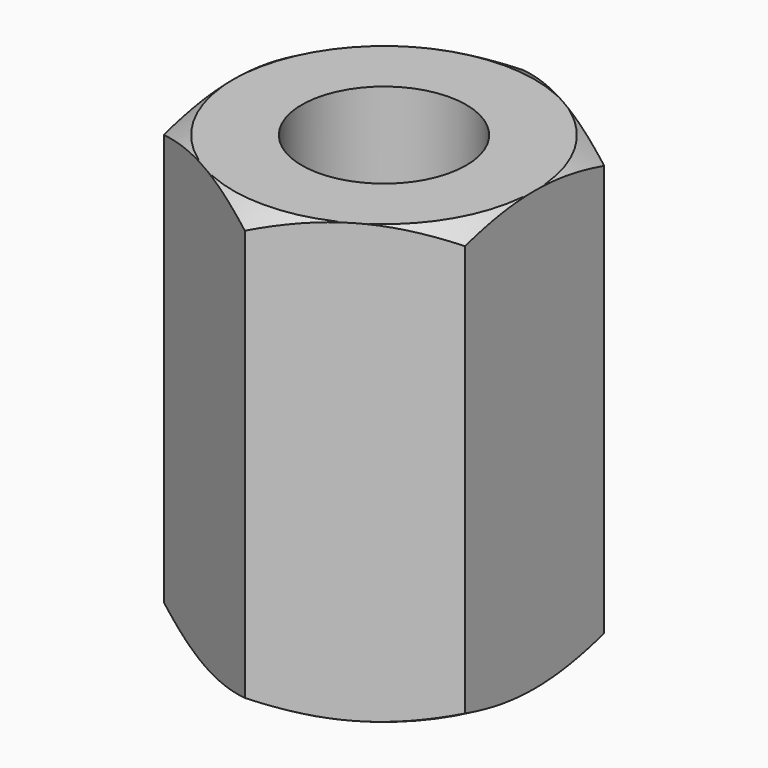
from build123d import *

# Parameters (mm, degrees)
F1_R     = 1.5
F2_DEPTH = 8
F5_R     = 1.25
F6_DEPTH = 6


with BuildPart() as f2:
    # F1 (on Top) → F2 (new body)
    with BuildSketch(Plane.XY):
        Polygon((2.75, 1.5877132403), (0, 3.1754264805), (-2.75, 1.5877132403), (-2.75, -1.5877132403), (0, -3.1754264805), (2.75, -1.5877132403), align=None)
        Circle(F1_R, mode=Mode.SUBTRACT)
    extrude(amount=F2_DEPTH)

    # F3 (on Front) → F4 (revolve, cut)
    with BuildSketch(Plane.XZ):
        Polygon((5.4806887836, 8), (2.75, 8), (5.4806887836, 6.4234360957), align=None)
        Polygon((5.4806887836, 1.5765639043), (2.75, 0), (5.4806887836, 0), align=None)
    revolve(axis=Axis((0, 0, 4), (0, 0, -1)), mode=Mode.SUBTRACT)


with BuildPart() as f6:
    # F5 (on Top) → F6 (new body)
    with BuildSketch(Plane.XY):
        Polygon((0, -2.8867513459), (2.5, -1.443375673), (2.5, 1.443375673), (0, 2.8867513459), (-2.5, 1.443375673), (-2.5, -1.443375673), align=None)
        Circle(F5_R, mode=Mode.SUBTRACT)
    extrude(amount=F6_DEPTH)

    # F7 (on Front) → F8 (revolve, cut)
    with BuildSketch(Plane.XZ):
        Polygon((4.3954963651, 6), (2.5, 6), (4.3954963651, 4.9056346634), align=None)
        Polygon((2.5, 0), (4.3954963651, 0), (4.3954963651, 1.0943653366), align=None)
    revolve(axis=Axis((0, 0, 3), (0, 0, -1)), mode=Mode.SUBTRACT)


solid = Compound([f2.part, f6.part])
